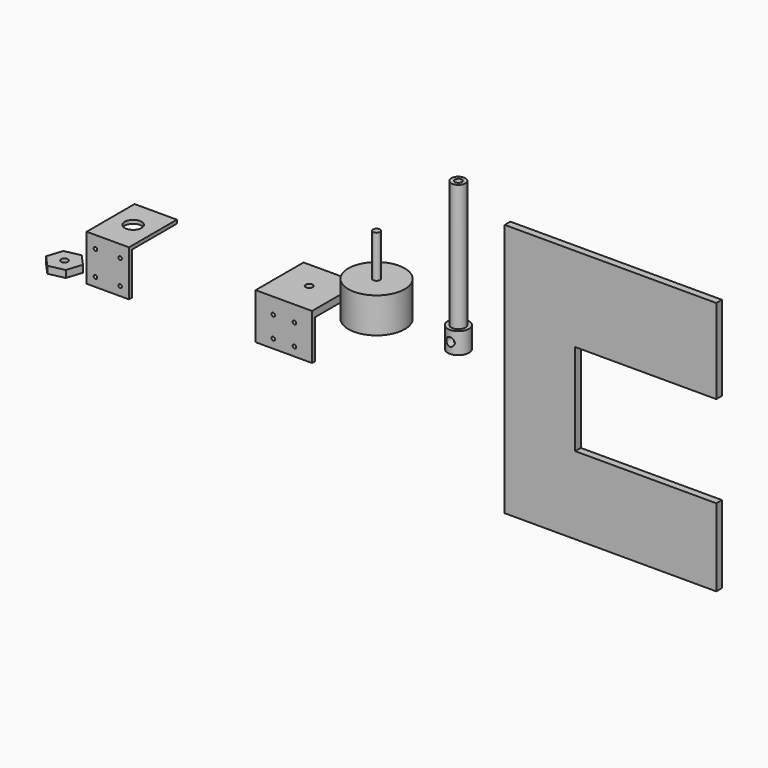
from build123d import *

# Parameters (mm, degrees)
F0_R      = 2.5
F1_DEPTH  = 15
F2_R      = 5
F2_R_2    = 2.5
F3_DEPTH  = 90
F5_R      = 3
F6_DEPTH  = 15.001
F0_R_2    = 20
F7_DEPTH  = 25
F8_R      = 2.5
F9_DEPTH  = 30
F0_W      = 40
F0_H      = 40
F10_DEPTH = 5
F11_W     = 40
F11_H     = 2.5
F12_DEPTH = 32.5
F14_DEPTH = 5
F0_W_2    = 30
F0_R_3    = 6
F16_DEPTH = 2.5
F17_W     = 30
F17_H     = 2.5
F18_DEPTH = 32.5
F19_DEPTH = 5
F20_R     = 1.25
F21_DEPTH = 2.5
F22_R     = 1.25
F23_DEPTH = 2.5


with BuildPart() as f1:
    # F0 (on Top) → F1 (new body)
    with BuildSketch(Plane.XY):
        with BuildLine():
            ThreePointArc((0, 7.5), (-5.3033008589, -5.3033008589), (7.5, 0))
            ThreePointArc((7.5, 0), (5.3033008589, 5.3033008589), (0, 7.5))
        make_face()
        Circle(F0_R, mode=Mode.SUBTRACT)
    extrude(amount=F1_DEPTH)

    # F2 (on face) → F3 (join)
    with BuildSketch(Plane.XY.offset(15)):
        Circle(F2_R)
        Circle(F2_R_2, mode=Mode.SUBTRACT)
    extrude(amount=F3_DEPTH)

    # F5 (on face) → F6 (cut, through all)
    with BuildSketch(Plane.XZ.offset(-7.5)):
        with Locations((0, 7.5)):
            Circle(F5_R)
    extrude(amount=F6_DEPTH, mode=Mode.SUBTRACT)


with BuildPart() as f7:
    # F0 (on Top) → F7 (new body)
    with BuildSketch(Plane.XY):
        with Locations((-57.9745993018, 0)):
            Circle(F0_R_2)
    extrude(amount=F7_DEPTH)

    # F8 (on face) → F9 (join)
    with BuildSketch(Plane.XY.offset(25)):
        with Locations((-57.9745993018, 0)):
            Circle(F8_R)
    extrude(amount=F9_DEPTH)


with BuildPart() as f10:
    # F0 (on Top) → F10 (new body)
    with BuildSketch(Plane.XY):
        with Locations((-105.7388707995, 0)):
            Rectangle(F0_W, F0_H)
        with Locations((-105.7388707995, 0)):
            Circle(F0_R, mode=Mode.SUBTRACT)
    extrude(amount=F10_DEPTH)

    # F11 (on face) → F12 (join)
    with BuildSketch(Plane.XY.offset(5)):
        with Locations((-105.7388707995, -21.25)):
            Rectangle(F11_W, F11_H)
    extrude(amount=-F12_DEPTH)

    # F20 (on face) → F21 (cut, through all)
    with BuildSketch(Plane(origin=(0, -20, 0), x_dir=(-1, 0, 0), z_dir=(0, 1, 0))):
        with Locations((98.2388707995, -6.25)):
            Circle(F20_R)
        with Locations((113.2388707995, -6.25)):
            Circle(F20_R)
        with Locations((113.2388707995, -21.25)):
            Circle(F20_R)
        with Locations((98.2388707995, -21.25)):
            Circle(F20_R)
    extrude(amount=-F21_DEPTH, mode=Mode.SUBTRACT)


with BuildPart() as f14:
    # F13 (on Front) → F14 (new body)
    with BuildSketch(Plane.XZ):
        Polygon((186.8768878281, 91.5050628316), (36.8768878281, 91.5050628316), (36.8768878281, -88.4949371684), (186.8768878281, -88.4949371684), (186.8768878281, -33.4949371684), (86.8768878281, -33.4949371684), (86.8768878281, 31.5050628316), (186.8768878281, 31.5050628316), align=None)
    extrude(amount=F14_DEPTH)


with BuildPart() as f16:
    # F0 (on Top) → F16 (new body)
    with BuildSketch(Plane.XY):
        with Locations((-230.5557584763, 0)):
            Rectangle(F0_W_2, F0_H)
        with Locations((-230.5557584763, 0)):
            Circle(F0_R_3, mode=Mode.SUBTRACT)
    extrude(amount=F16_DEPTH)

    # F17 (on face) → F18 (join)
    with BuildSketch(Plane.XY.offset(2.5)):
        with Locations((-230.5557584763, -21.25)):
            Rectangle(F17_W, F17_H)
    extrude(amount=-F18_DEPTH)

    # F22 (on face) → F23 (cut, through all)
    with BuildSketch(Plane(origin=(0, -20, 0), x_dir=(-1, 0, 0), z_dir=(0, 1, 0))):
        with Locations((221.8057584763, -6.25)):
            Circle(F22_R)
        with Locations((221.8057584763, -23.75)):
            Circle(F22_R)
        with Locations((239.3057584763, -23.75)):
            Circle(F22_R)
        with Locations((239.3057584763, -6.25)):
            Circle(F22_R)
    extrude(amount=-F23_DEPTH, mode=Mode.SUBTRACT)


with BuildPart() as f19:
    # F0 (on Top) → F19 (new body)
    with BuildSketch(Plane.XY):
        Polygon((-222.9001823011, -69.3075905842), (-219.3971571383, -58.4452201324), (-227.0527333135, -49.9803261255), (-238.2113346515, -52.3778025704), (-241.7143598142, -63.2401730222), (-234.058783639, -71.7050670291), align=None)
        with Locations((-230.5557584763, -60.8426965773)):
            Circle(F0_R, mode=Mode.SUBTRACT)
    extrude(amount=F19_DEPTH)


solid = Compound([f1.part, f7.part, f10.part, f14.part, f16.part, f19.part])
